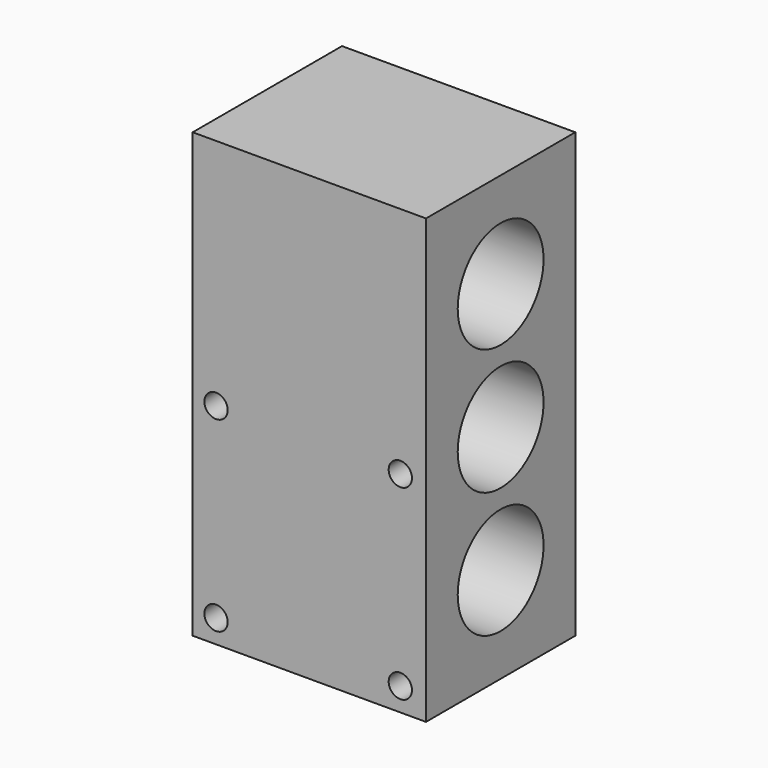
from build123d import *

# Parameters (mm, degrees)
F0_W      = 50
F0_H      = 95
F1_DEPTH  = 40
F2_R      = 2.5
F3_DEPTH  = 18
F4_R      = 11.5
F5_DEPTH  = 20
F7_R      = 11.5
F8_DEPTH  = 50.001
F9_R      = 3
F10_DEPTH = 25


# Not quite as in the source:
# - a pattern or mirror of a feature is missing from the dataset's text; its kind, count and spacing are read off the source's solid


with BuildPart() as f1:
    # F0 (on Front) → F1 (new body)
    with BuildSketch(Plane.XZ):
        with Locations((25, 47.5)):
            Rectangle(F0_W, F0_H)
    extrude(amount=F1_DEPTH)

    # F2 (on face) → F3 (cut)
    with BuildSketch(Plane.XZ.offset(40)):
        with Locations((5, 5)):
            Circle(F2_R)
        with Locations((44.5, 5)):
            Circle(F2_R)
        with Locations((5, 45)):
            Circle(F2_R)
        with Locations((44.5, 45)):
            Circle(F2_R)
    extrude(amount=-F3_DEPTH, mode=Mode.SUBTRACT)

    # F4 (on face) → F5 (cut)
    with BuildSketch(Plane(origin=(0, 0, 0), x_dir=(0, -1, 0), z_dir=(-1, 0, 0))):
        with Locations((20, 74.5)):
            Circle(F4_R)
        with Locations((20, 20.5)):
            Circle(F4_R)
    f5 = extrude(amount=-F5_DEPTH, mode=Mode.SUBTRACT)

    # F5_copies: F5 across plane
    add(f5.mirror(Plane(origin=(25, 0, 0), x_dir=(0, 0, 1), z_dir=(1, 0, 0))), mode=Mode.SUBTRACT)

    # F7 (on face) → F8 (cut, through all)
    with BuildSketch(Plane(origin=(0, 0, 0), x_dir=(0, -1, 0), z_dir=(-1, 0, 0))):
        with Locations((20, 47.5)):
            Circle(F7_R)
    extrude(amount=-F8_DEPTH, mode=Mode.SUBTRACT)

    # F9 (on face) → F10 (cut)
    with BuildSketch(Plane(origin=(0, 0, 0), x_dir=(0, -1, 0), z_dir=(-1, 0, 0))):
        with Locations((32.5, 57.5)):
            Circle(F9_R)
        with Locations((7.5, 37.5)):
            Circle(F9_R)
    extrude(amount=-F10_DEPTH, mode=Mode.SUBTRACT)


solid = f1.part
